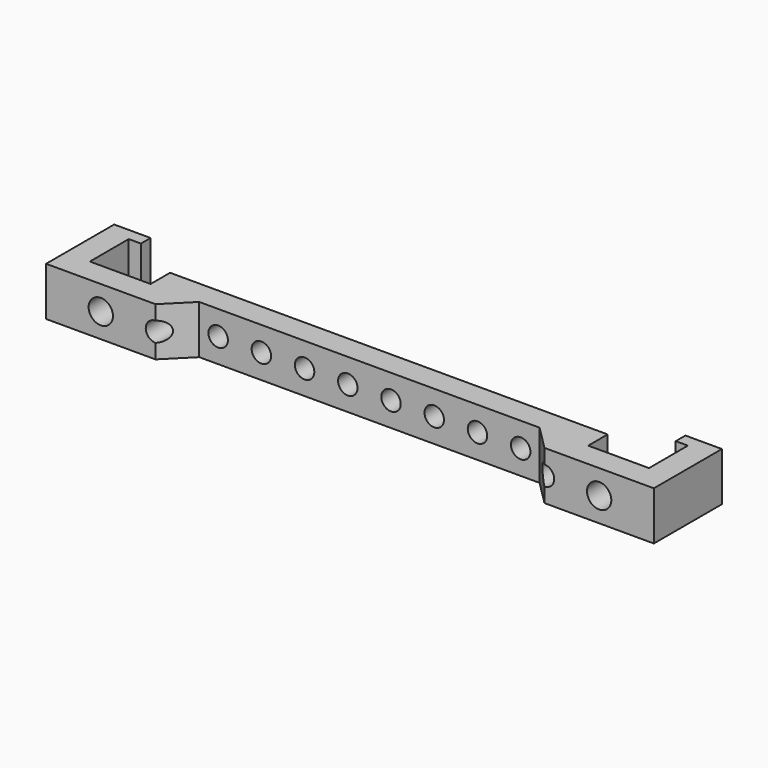
from build123d import *

# Parameters (mm, degrees)
F0_W     = 16
F0_H     = 2
F0_W_2   = 2
F0_W_3   = 1
F0_H_2   = 1
F1_DEPTH = 4
F2_SIZE  = 1.99999
F3_R     = 1
F4_DEPTH = 2
F5_R     = 0.8008995453
F6_DEPTH = 5


# Not quite as in the source:
# - a fillet or chamfer is up to 0.001 mm smaller than in the source, because OpenCascade refuses the exact size


with BuildPart() as f1:
    # F0 (on Top) → F1 (new body)
    with BuildSketch(Plane.XY):
        with Locations((33, -4)):
            Rectangle(F0_W, F0_H)
        with Locations((17, -4)):
            Rectangle(F0_W, F0_H)
        Polygon((48, -5), (43, -5), (43, -7), (50, -7), (50, -5), align=None)
        with Locations((42, -6)):
            Rectangle(F0_W_2, F0_H)
        Polygon((2, -5), (0, -5), (0, -7), (7, -7), (7, -5), align=None)
        Polygon((2, 0), (0, 0), (0, -5), (2, -5), (2, -1), align=None)
        with Locations((47.5, -0.5)):
            Rectangle(F0_W_3, F0_H_2)
        with Locations((8, -4)):
            Rectangle(F0_W_2, F0_H)
        with Locations((8, -6)):
            Rectangle(F0_W_2, F0_H)
        with Locations((2.5, -0.5)):
            Rectangle(F0_W_3, F0_H_2)
        with Locations((42, -4)):
            Rectangle(F0_W_2, F0_H)
        Polygon((48, -1), (48, -5), (50, -5), (50, 0), (48, 0), align=None)
    extrude(amount=F1_DEPTH)

    # F2 (size 2 in the source; OpenCascade refuses exactly that, so slightly less here)
    f2_edges = [f1.edges().sort_by_distance(p)[0] for p in [
        (41, -5, 2),
        (9, -5, 2),
    ]]
    chamfer(f2_edges, length=F2_SIZE)

    # F3 (on face) → F4 (cut)
    with BuildSketch(Plane(origin=(0, -5, 0), x_dir=(-1, 0, 0), z_dir=(0, 1, 0))):
        with Locations((-4.5, 2)):
            Circle(F3_R)
        with Locations((-45.5, 2)):
            Circle(F3_R)
    extrude(amount=-F4_DEPTH, mode=Mode.SUBTRACT)

    # F5 (on face) → F6 (cut)
    with BuildSketch(Plane(origin=(0, -3, 0), x_dir=(-1, 0, 0), z_dir=(0, 1, 0))):
        with Locations((-16.1111111111, 2)):
            Circle(F5_R)
        with Locations((-9, 2)):
            Circle(F5_R)
        with Locations((-12.5555555556, 2)):
            Circle(F5_R)
        with Locations((-19.6666666667, 2)):
            Circle(F5_R)
        with Locations((-23.2222222222, 2)):
            Circle(F5_R)
        with Locations((-26.7777777778, 2)):
            Circle(F5_R)
        with Locations((-30.3333333333, 2)):
            Circle(F5_R)
        with Locations((-33.8888888889, 2)):
            Circle(F5_R)
        with Locations((-37.4444444444, 2)):
            Circle(F5_R)
        with Locations((-41, 2)):
            Circle(F5_R)
    extrude(amount=-F6_DEPTH, mode=Mode.SUBTRACT)


solid = f1.part
